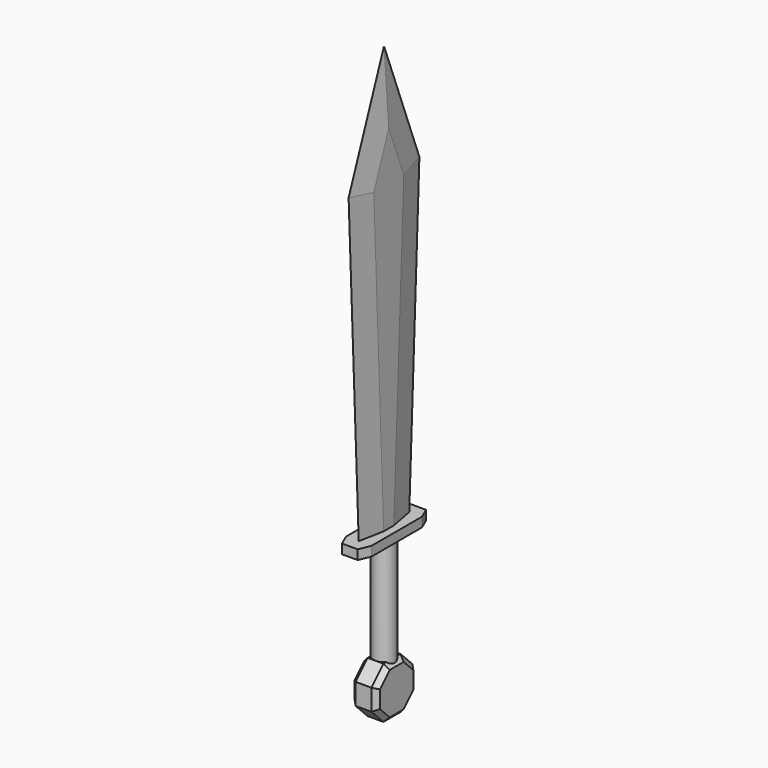
from build123d import *

# Parameters (mm, degrees)
F1_DEPTH  = 3.81
F2_SIZE2  = 3.81
F2_SIZE   = 20.32
F3_SIZE2  = 3.80999
F3_SIZE   = 20.31999
F5_DEPTH  = 7.62
F6_R      = 8.5322450092
F7_DEPTH  = 83.82
F9_R      = 8.5322450092
F10_DEPTH = 25.4
F11_DEPTH = 10.16
F12_SIZE  = 3.81


# Not quite as in the source:
# - a fillet or chamfer is up to 0.001 mm smaller than in the source, because OpenCascade refuses the exact size
# - ends of sketch curves that miss each other by under 0.0002 mm in the source are joined


with BuildPart() as f1:
    # F0 (on Right) → F1 (new body, symmetric)
    with BuildSketch(Plane.YZ):
        Polygon((-25.4, 0), (0, 0), (0, 82.3990235604), (0, 247.1720576286), (-35.56, 247.1720576286), align=None)
        Polygon((0, 82.3990235604), (0, 0), (25.4, 0), (35.56, 247.1720576286), (0, 247.1720576286), align=None)
        Polygon((0, 340.030759573), (0, 247.1720576286), (35.56, 247.1720576286), align=None)
        Polygon((-35.56, 247.1720576286), (0, 247.1720576286), (0, 340.030759573), align=None)
    extrude(amount=F1_DEPTH, both=True)

    # F2
    f2_edges = [f1.edges().sort_by_distance(p)[0] for p in [
        (3.81, -30.48, 123.586029),
        (3.81, -17.78, 293.601409),
        (3.81, 17.78, 293.601409),
        (3.81, 30.48, 123.586029),
    ]]
    f2_side = f1.faces().sort_by_distance((3.81, 0, 156.997019))[0]
    chamfer(f2_edges, length=F2_SIZE, length2=F2_SIZE2, reference=f2_side)

    # F3 (size 20.32 and 3.81 in the source; OpenCascade refuses exactly that, so slightly less here)
    f3_edges = [f1.edges().sort_by_distance(p)[0] for p in [
        (-3.81, -30.48, 123.586029),
        (-3.81, -17.78, 293.601409),
        (-3.81, 30.48, 123.586029),
        (-3.81, 17.78, 293.601409),
    ]]
    f3_side = f1.faces().sort_by_distance((-3.81, 0, 156.997019))[0]
    chamfer(f3_edges, length=F3_SIZE, length2=F3_SIZE2, reference=f3_side)


with BuildPart() as f5:
    # F4 (on face) → F5 (new body)
    with BuildSketch(Plane(origin=(0, 0, 0), x_dir=(1, 0, 0), z_dir=(0, 0, -1))):
        Polygon((6.35, 34.3802462), (-6.35, 34.3802462), (-10.16, 25.3999900789), (-10.16, -9.9211e-06), (0, 0), (10.16, -9.9211e-06), (10.16, 25.3999900789), align=None)
        Polygon((0, 0), (-10.16, -9.9211e-06), (-10.16, -25.4000099211), (-6.35, -34.3802660421), (6.35, -34.3802660421), (10.16, -25.4000099211), (10.16, -9.9211e-06), align=None)
    extrude(amount=F5_DEPTH)


with BuildPart() as f7:
    # F6 (on face) → F7 (new body)
    with BuildSketch(Plane(origin=(0, 0, -7.62), x_dir=(1, 0, 0), z_dir=(0, 0, -1))):
        Circle(F6_R)
    extrude(amount=F7_DEPTH)

    # F9 (on face) → F10 (join)
    with BuildSketch(Plane(origin=(0, 0, -91.44), x_dir=(1, 0, 0), z_dir=(0, 0, -1))):
        Circle(F9_R)
    extrude(amount=F10_DEPTH)


with BuildPart() as f11:
    # F8 (on Right) → F11 (new body, symmetric)
    with BuildSketch(Plane.YZ):
        Polygon((20.5986616187, -103.5064166095), (8.5322450092, -91.44), (0, -91.44), (-8.5322450092, -91.44), (-20.5986616187, -103.5064166095), (-20.5986616187, -120.5709066278), (-8.5322450092, -132.6373232373), (8.5322450092, -132.6373232373), (20.5986616187, -120.5709066278), align=None)
    extrude(amount=F11_DEPTH, both=True)

    # F12
    f12_edges = [f11.edges().sort_by_distance(p)[0] for p in [
        (10.16, 20.598662, -112.038662),
        (10.16, 14.565453, -97.473208),
        (10.16, 0, -91.44),
        (10.16, 14.565453, -126.604115),
        (10.16, 0, -132.637323),
        (10.16, -14.565453, -126.604115),
        (10.16, -14.565453, -97.473208),
        (10.16, -20.598662, -112.038662),
        (-10.16, -20.598662, -112.038662),
        (-10.16, -14.565453, -97.473208),
        (-10.16, -14.565453, -126.604115),
        (-10.16, 0, -132.637323),
        (-10.16, 0, -91.44),
        (-10.16, 14.565453, -97.473208),
        (-10.16, 20.598662, -112.038662),
        (-10.16, 14.565453, -126.604115),
    ]]
    chamfer(f12_edges, length=F12_SIZE)


solid = Compound([f1.part, f5.part, f7.part, f11.part])
